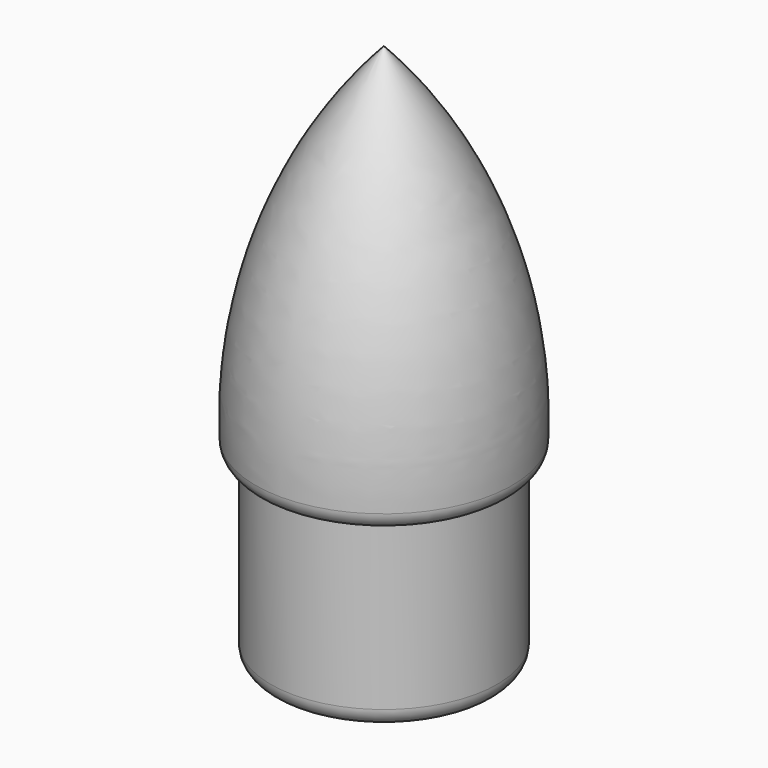
from build123d import *


# Not quite as in the source:
# - a fillet or chamfer that OpenCascade refuses, or shapes differently, is made with other operations: its cross-section is extruded or revolved along the edge and cut away or added


with BuildPart() as f1:
    # F0 (on Right) → F1 (revolve)
    with BuildSketch(Plane.YZ):
        with BuildLine():
            Line((-31.75, 0), (0, 0))
            Line((0, 0), (0, 152.4))
            ThreePointArc((0, 152.4), (-28.4861105744, 105.3337323133), (-35.75, 50.8))
            Line((-35.75, 50.8), (-31.75, 50.8))
            Line((-31.75, 50.8), (-31.75, 0))
        make_face()
    revolve(axis=Axis((0, 0, 76.2), (0, 0, 1)))

    # F2: fillet of radius 5.08 on 2 edges, made by hand

    # F2_s1 → F2_t2 (revolve, cut)
    with BuildSketch(Plane.YZ):
        with BuildLine():
            ThreePointArc((-36.0182250356, 55.6244324438), (-34.7465352987, 52.4492219117), (-31.75, 50.8))
            Line((-31.75, 50.8), (-35.75, 50.8))
            ThreePointArc((-35.75, 50.8), (-35.9057734532, 53.2110119341), (-36.0182250356, 55.6244324438))
        make_face()
    revolve(axis=Axis((0, 0, 50.8), (0, 0, 1)), mode=Mode.SUBTRACT)

    # F2_s3 → F2_t4 (revolve, cut)
    with BuildSketch(Plane.YZ):
        with BuildLine():
            ThreePointArc((-31.75, 5.08), (-30.2621024484, 1.4878975516), (-26.67, 0))
            Line((-26.67, 0), (-31.75, 0))
            Line((-31.75, 0), (-31.75, 5.08))
        make_face()
    revolve(axis=Axis((0, 0, 0), (0, 0, 1)), mode=Mode.SUBTRACT)


solid = f1.part
